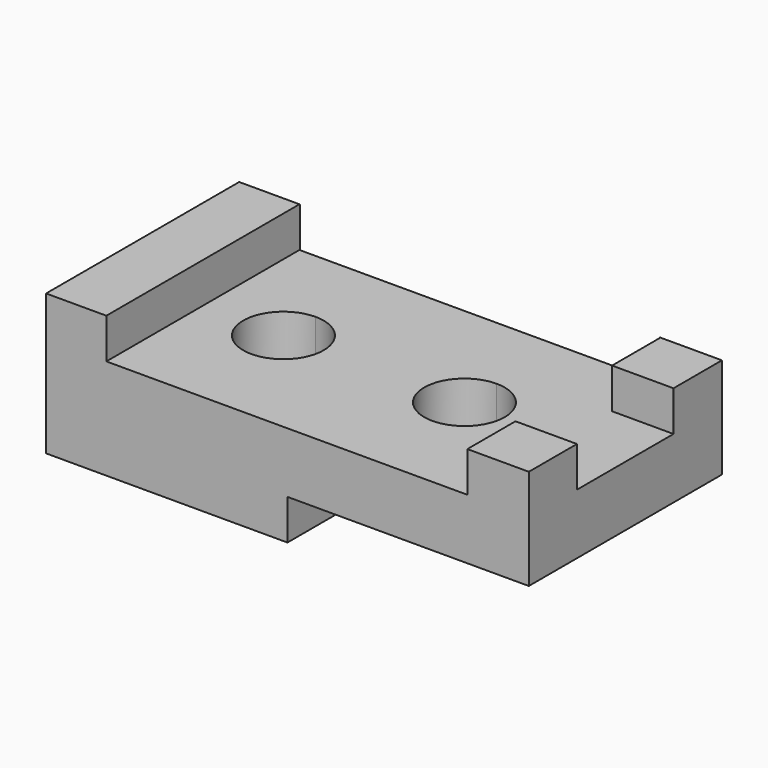
from build123d import *

# Parameters (mm, degrees)
F0_W      = 60
F0_H      = 60
F1_DEPTH  = 10
F2_W      = 60
F2_H      = 60
F3_DEPTH  = 25
F5_DEPTH  = 51.5
F7_DEPTH  = 10
F8_W      = 19.9074504152
F8_H      = 1.7359393835
F8_W_2    = 45
F8_W_3    = 24.514567852
F9_DEPTH  = 10
F10_W     = 2.977065742
F10_H     = 29.9195116386
F11_DEPTH = 10


with BuildPart() as f1:
    # F0 (on Top) → F1 (new body)
    with BuildSketch(Plane.XY):
        Rectangle(F0_W, F0_H)
    extrude(amount=F1_DEPTH)

    # F2 (on face) → F3 (join)
    with BuildSketch(Plane.XY.offset(10)):
        Rectangle(F2_W, F2_H)
        with Locations((60, 0)):
            Rectangle(F2_W, F2_H)
    extrude(amount=F3_DEPTH)

    # F4 (on face) → F5 (cut)
    with BuildSketch(Plane.XY.offset(35)):
        with BuildLine():
            ThreePointArc((60, 0), (57.0710678119, 7.0710678119), (50, 10))
            ThreePointArc((50, 10), (42.9289321881, -7.0710678119), (60, 0))
        make_face()
        with BuildLine():
            ThreePointArc((15, 0), (12.0710678119, 7.0710678119), (5, 10))
            ThreePointArc((5, 10), (-2.0710678119, -7.0710678119), (15, 0))
        make_face()
    extrude(amount=-F5_DEPTH, mode=Mode.SUBTRACT)

    # F6 (on face) → F7 (cut)
    with BuildSketch(Plane.XY.offset(35)):
        Polygon((5, 29.9537748588), (-15.0160359405, 29.9537740648), (-15.0160359405, -30), (74.7204658659, -30), (74.7204658659, -15.0462223754), (89.7204658659, -15.0462223754), (89.7204658659, 14.9537776246), (74.7204658659, 14.9537776246), (74.7204658659, 29.9537776246), (50, 29.953776644), align=None)
        with BuildLine():
            ThreePointArc((15, 0), (-2.0710678119, -7.0710678119), (5, 10))
            ThreePointArc((5, 10), (12.0710678119, 7.0710678119), (15, 0))
        make_face(mode=Mode.SUBTRACT)
        with BuildLine():
            ThreePointArc((60, 0), (42.9289321881, -7.0710678119), (50, 10))
            ThreePointArc((50, 10), (57.0710678119, 7.0710678119), (60, 0))
        make_face(mode=Mode.SUBTRACT)
    extrude(amount=-F7_DEPTH, mode=Mode.SUBTRACT)

    # F8 (on face) → F9 (cut)
    with BuildSketch(Plane.XY.offset(35)):
        with Locations((-4.9537252076, 29.1320303082)):
            Rectangle(F8_W, F8_H)
        with Locations((27.5, 29.1320303082)):
            Rectangle(F8_W_2, F8_H)
        with Locations((62.257283926, 29.1320303082)):
            Rectangle(F8_W_3, F8_H)
    extrude(amount=-F9_DEPTH, mode=Mode.SUBTRACT)

    # F10 (on face) → F11 (cut)
    with BuildSketch(Plane.XY.offset(35)):
        with Locations((91.1140106618, -0.0397800468)):
            Rectangle(F10_W, F10_H)
    extrude(amount=-F11_DEPTH, mode=Mode.SUBTRACT)


solid = f1.part
